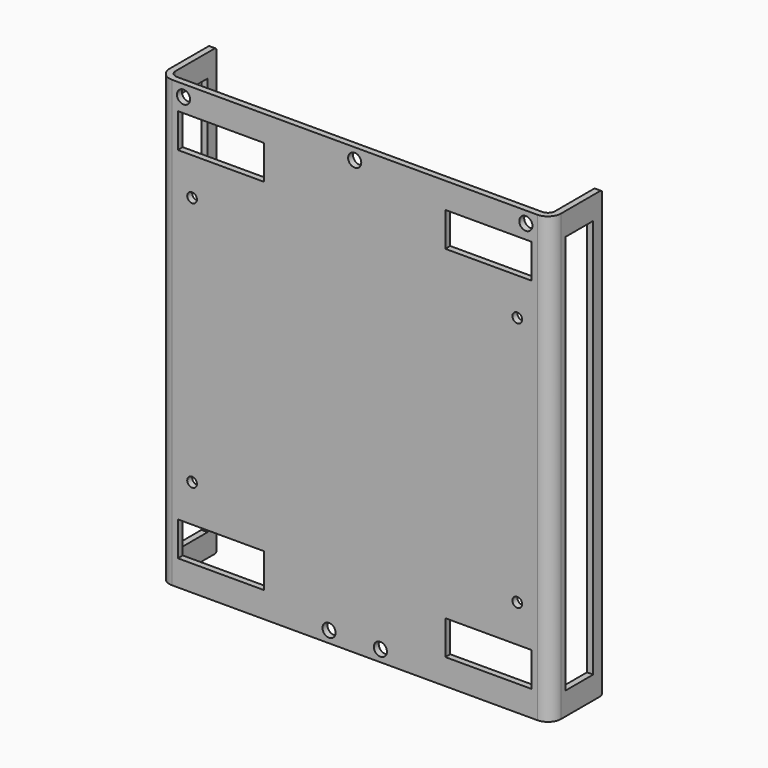
from build123d import *

# Parameters (mm, degrees)
F1_DEPTH = 123.825
F2_W     = 9.525
F2_H     = 111.125
F3_DEPTH = 108.98632
F4_R     = 3.69316
F5_R     = 1.98374
F6_R     = 1.8288
F6_W     = 24
F6_H     = 9.5329248
F6_R_2   = 1.35255
F7_DEPTH = 248
F8_R     = 0.762


# Not quite as in the source:
# - an extrude ends at something that could not be found from the text; its depth is read off the source's solid


with BuildPart() as f1:
    # F0 (on Top) → F1 (new body)
    with BuildSketch(Plane.XY):
        Polygon((0, 16.27124), (0, 0), (-105.56748, 0), (-105.56748, 16.27124), (-107.2769, 16.27124), (-107.2769, -1.70942), (1.70942, -1.70942), (1.70942, 16.27124), align=None)
    extrude(amount=F1_DEPTH)

    # F2 (on face) → F3 (cut, through all)
    with BuildSketch(Plane.YZ.offset(1.70942)):
        with Locations((8.33374, 61.9125)):
            Rectangle(F2_W, F2_H)
    extrude(amount=-F3_DEPTH, mode=Mode.SUBTRACT)

    # F4
    f4_edges = [f1.edges().sort_by_distance(p)[0] for p in [
        (1.70942, -1.70942, 61.9125),
        (-107.2769, -1.70942, 61.9125),
    ]]
    fillet(f4_edges, radius=F4_R)

    # F5
    f5_edges = [f1.edges().sort_by_distance(p)[0] for p in [
        (0, 0, 61.9125),
        (-105.56748, 0, 61.9125),
    ]]
    fillet(f5_edges, radius=F5_R)

    # F6 (on face) → F7 (cut, through all)
    with BuildSketch(Plane.XZ.offset(1.70942)):
        with Locations((-52.78374, 120.65)):
            Circle(F6_R)
        with Locations((-5.15874, 120.65)):
            Circle(F6_R)
        with Locations((-100.40874, 120.65)):
            Circle(F6_R)
        with Locations((-45.63999, 3.175)):
            Circle(F6_R)
        with Locations((-59.92749, 3.175)):
            Circle(F6_R)
        with Locations((-89.99624, 111.9147876)):
            Rectangle(F6_W, F6_H)
        with Locations((-89.99624, 11.9102124)):
            Rectangle(F6_W, F6_H)
        with Locations((-15.57124, 111.9147876)):
            Rectangle(F6_W, F6_H)
        with Locations((-15.57124, 11.9102124)):
            Rectangle(F6_W, F6_H)
        with Locations((-98.02749, 96.7528672)):
            Circle(F6_R_2)
        with Locations((-98.02749, 27.0721328)):
            Circle(F6_R_2)
        with Locations((-7.53999, 27.0721328)):
            Circle(F6_R_2)
        with Locations((-7.53999, 96.7528672)):
            Circle(F6_R_2)
    extrude(amount=-F7_DEPTH, mode=Mode.SUBTRACT)

    # F8
    f8_edges = [f1.edges().sort_by_distance(p)[0] for p in [
        (-106.42219, 16.27124, 123.825),
        (0.85471, 16.27124, 123.825),
        (0.85471, 16.27124, 0),
        (-106.42219, 16.27124, 0),
    ]]
    fillet(f8_edges, radius=F8_R)


solid = f1.part
